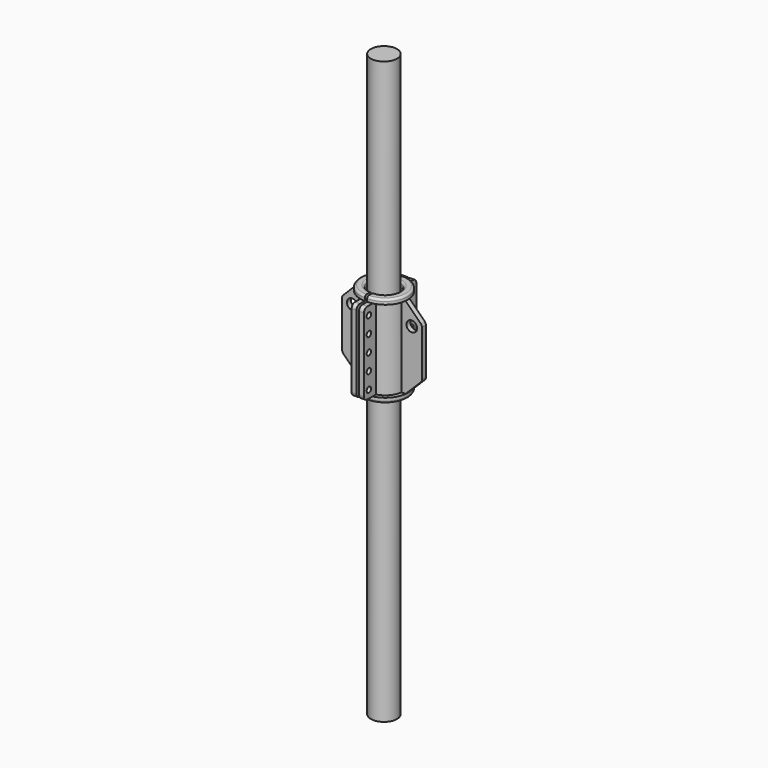
from build123d import *

# Parameters (mm, degrees)
F1_DEPTH      = 200
F3_D          = 13.5
F4_SIZE       = 40
F6_R          = 10
F8_DEPTH      = 12
F11_DEPTH     = 12
F12_D         = 26
F13_R         = 10
F14_T2_ANGLE  = 180
F14_T4_ANGLE  = 180
F14_T6_ANGLE  = 206.0854190728
F14_T8_ANGLE  = 206.0854190728
F14_T10_ANGLE = 220.9913728288
F14_T12_ANGLE = 220.9913728288
F17_R         = 32
F18_DEPTH     = 710


# Not quite as in the source:
# - a fillet or chamfer that OpenCascade refuses, or shapes differently, is made with other operations: its cross-section is extruded or revolved along the edge and cut away or added


with BuildPart() as f1:
    # F0 (on Top) → F1 (new body)
    with BuildSketch(Plane.XY):
        with BuildLine():
            ThreePointArc((0, 37), (37, 0), (0, -37))
            Line((0, -37), (0, -45))
            ThreePointArc((0, -45), (6.0550656562, -44.5907633922), (12, -43.3704968844))
            ThreePointArc((12, -43.3704968844), (33.9113218085, -29.5807750609), (44.598206242, -6))
            ThreePointArc((44.598206242, -6), (45, 0), (44.598206242, 6))
            ThreePointArc((44.598206242, 6), (33.9113218085, 29.5807750609), (12, 43.3704968844))
            ThreePointArc((12, 43.3704968844), (6.0550656562, 44.5907633922), (0, 45))
            Line((0, 45), (0, 37))
        make_face()
        with BuildLine():
            Line((0, 80), (0, 45))
            ThreePointArc((0, 45), (6.0550656562, 44.5907633922), (12, 43.3704968844))
            Line((12, 43.3704968844), (12, 80))
            Line((12, 80), (0, 80))
        make_face()
        with BuildLine():
            ThreePointArc((44.598206242, 6), (45, 0), (44.598206242, -6))
            Line((44.598206242, -6), (94.598206242, -6))
            Line((94.598206242, -6), (94.598206242, 6))
            Line((94.598206242, 6), (44.598206242, 6))
        make_face()
        with BuildLine():
            ThreePointArc((12, -43.3704968844), (6.0550656562, -44.5907633922), (0, -45))
            Line((0, -45), (0, -80))
            Line((0, -80), (12, -80))
            Line((12, -80), (12, -43.3704968844))
        make_face()
    extrude(amount=F1_DEPTH)

    # F3 (through all)
    with Locations(Plane(origin=(0, 0, 0), x_dir=(0, 1, 0), z_dir=(-1, 0, 0))):
        with Locations((-65, -179), (-64.9707055397, -139.0000107271), (-64.9414110793, -99.0000214541), (-64.912116619, -59.0000321812), (-64.8828221586, -19.0000429083), (65, -179), (64.9707055397, -139.0000107271), (64.9414110793, -99.0000214541), (64.912116619, -59.0000321812), (64.8828221586, -19.0000429083)):
            Hole(F3_D / 2)

    # F4
    f4_edges = [f1.edges().sort_by_distance(p)[0] for p in [
        (94.598206, 0, 200),
        (94.598206, 0, 0),
    ]]
    chamfer(f4_edges, length=F4_SIZE)

    # F6
    f6_edges = [f1.edges().sort_by_distance(p)[0] for p in [
        (94.598206, 0, 160),
        (94.598206, 0, 40),
    ]]
    fillet(f6_edges, radius=F6_R)

    # F7 (on Top) → F8 (join)
    with BuildSketch(Plane.XY):
        with BuildLine():
            Line((0, -35), (0, -55))
            ThreePointArc((0, -55), (55, 0), (0, 55))
            Line((0, 55), (0, 35))
            ThreePointArc((0, 35), (35, 0), (0, -35))
        make_face()
    extrude(amount=-F8_DEPTH)

    # F10 (on offset) → F11 (join)
    with BuildSketch(Plane.XY.offset(200)):
        with BuildLine():
            Line((0, -35), (0, -55))
            ThreePointArc((0, -55), (55, 0), (0, 55))
            Line((0, 55), (0, 35))
            ThreePointArc((0, 35), (35, 0), (0, -35))
        make_face()
    extrude(amount=F11_DEPTH)

    # F12 (through all)
    with Locations(Plane(origin=(0, 6, 0), x_dir=(-1, 0, 0), z_dir=(0, 1, 0))):
        with Locations((-69.598206242, 150)):
            Hole(F12_D / 2)

    # F13
    f13_edges = [f1.edges().sort_by_distance(p)[0] for p in [
        (6, -80, 200),
        (6, 80, 200),
        (6, 80, 0),
        (6, -80, 0),
    ]]
    fillet(f13_edges, radius=F13_R)

    # F14: fillet of radius 5 on 6 edges, made by hand

    # F14_s1 → F14_t2 (revolve)
    with BuildSketch(Plane.YZ):
        with BuildLine():
            ThreePointArc((35, 200), (36.472135955, 198.2360679775), (37, 196))
            Line((37, 196), (37, 200))
            Line((37, 200), (35, 200))
        make_face()
    revolve(axis=Axis((0, 0, 200), (0, 0, -1)), revolution_arc=F14_T2_ANGLE)

    # F14_s3 → F14_t4 (revolve)
    with BuildSketch(Plane.YZ):
        with BuildLine():
            ThreePointArc((37, 4), (36.472135955, 1.7639320225), (35, 0))
            Line((35, 0), (37, 0))
            Line((37, 0), (37, 4))
        make_face()
    revolve(axis=Axis((0, 0, 0), (0, 0, -1)), revolution_arc=F14_T4_ANGLE)

    # F14_s5 → F14_t6 (revolve, cut)
    with BuildSketch(Plane(origin=(0, 0, 0), x_dir=(0, 0, 1), z_dir=(-0.9742021106, 0.2256773087, 0))):
        with BuildLine():
            ThreePointArc((-7, -55), (-10.5355339059, -53.5355339059), (-12, -50))
            Line((-12, -50), (-12, -55))
            Line((-12, -55), (-7, -55))
        make_face()
    revolve(axis=Axis((0, 0, -12), (0, 0, 1)), revolution_arc=F14_T6_ANGLE, mode=Mode.SUBTRACT)

    # F14_s7 → F14_t8 (revolve, cut)
    with BuildSketch(Plane(origin=(0, 0, 0), x_dir=(0, 0, 1), z_dir=(-0.9742021106, 0.2256773087, 0))):
        with BuildLine():
            ThreePointArc((207, -55), (210.5355339059, -53.5355339059), (212, -50))
            Line((212, -50), (212, -55))
            Line((212, -55), (207, -55))
        make_face()
    revolve(axis=Axis((0, 0, 212), (0, 0, 1)), revolution_arc=F14_T8_ANGLE, mode=Mode.SUBTRACT)

    # F14_s9 → F14_t10 (revolve, cut)
    with BuildSketch(Plane(origin=(0, 0, 0), x_dir=(0, 0, 1), z_dir=(-0.9366985524, -0.3501368617, 0))):
        with BuildLine():
            ThreePointArc((212, 40), (210.5355339059, 36.4644660941), (207, 35))
            Line((207, 35), (212, 35))
            Line((212, 35), (212, 40))
        make_face()
    revolve(axis=Axis((0, 0, 212), (0, 0, -1)), revolution_arc=F14_T10_ANGLE, mode=Mode.SUBTRACT)

    # F14_s11 → F14_t12 (revolve, cut)
    with BuildSketch(Plane(origin=(0, 0, 0), x_dir=(0, 0, 1), z_dir=(-0.9366985524, -0.3501368617, 0))):
        with BuildLine():
            ThreePointArc((-7, 35), (-10.5355339059, 36.4644660941), (-12, 40))
            Line((-12, 40), (-12, 35))
            Line((-12, 35), (-7, 35))
        make_face()
    revolve(axis=Axis((0, 0, -12), (0, 0, -1)), revolution_arc=F14_T12_ANGLE, mode=Mode.SUBTRACT)


with BuildPart() as f16_1:
    # F16: instance of F1
    add(f1.part.mirror(Plane.YZ.offset(-3)))


with BuildPart() as f18:
    # F17 (on Top) → F18 (new body, symmetric)
    with BuildSketch(Plane.XY):
        with Locations((-3.1377882697, 0)):
            Circle(F17_R)
    extrude(amount=F18_DEPTH, both=True)


solid = Compound([f1.part, f16_1.part, f18.part])
